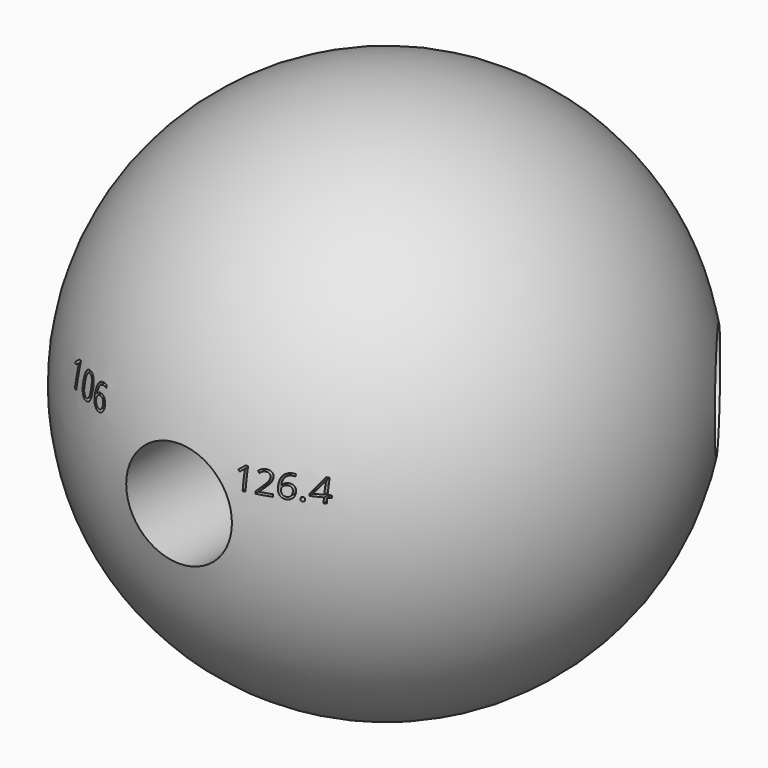
from build123d import *

# Parameters (mm, degrees)
F4_R           = 3.175
F5_DEPTH       = 25.4
F6_ANGLE       = -106
F7_ANGLE       = -127.6
F9_TEXT_SIZE   = 1.9675951787
F9_TEXT_SIZE_2 = 1.7945879437
F10_DEPTH      = 6.35
F12_TEXT_SIZE  = 1.7603325735
F13_DEPTH      = 5.969


# Not quite as in the source:
# - Text() gives the source's letters only with a copy of the font that has no kerning and outlines rounded to 1/6400 em; it was checked with that copy


with BuildPart() as f2:
    # F1 (on Top) → F2 (revolve)
    with BuildSketch(Plane.XY):
        with BuildLine():
            Line((0, -15.875), (0, 15.875))
            ThreePointArc((0, 15.875), (-15.875, 0), (0, -15.875))
        make_face()
    revolve(axis=Axis((0, 0, 0), (0, -1, 0)))

    # F9 (on offset) → F10 (cut)
    with BuildSketch(Plane.XZ.offset(19.05)):
        with Locations((-8.4282197058, 2.6850800496)):
            Text('106', F9_TEXT_SIZE, font='Open Sans', text_align=(TextAlign.LEFT, TextAlign.BOTTOM))
        with Locations((3.1687500887, 1.7594042001)):
            Text('126.4', F9_TEXT_SIZE_2, font='Open Sans', text_align=(TextAlign.LEFT, TextAlign.BOTTOM))
    extrude(amount=-F10_DEPTH, mode=Mode.SUBTRACT)

    # F12 (on offset) → F13 (cut)
    with BuildSketch(Plane(origin=(-18.3120353076, 5.2508916283, 0), x_dir=(-0.2756373558, -0.9612616959, 0), z_dir=(-0.9612616959, 0.2756373558, 0))):
        with Locations((-8.1116128713, 1.9357244018)):
            Text('127.6', F12_TEXT_SIZE, font='Open Sans', text_align=(TextAlign.LEFT, TextAlign.BOTTOM))
    extrude(amount=-F13_DEPTH, mode=Mode.SUBTRACT)


with BuildPart() as f5:
    # F4 (on offset) → F5 (new body)
    with BuildSketch(Plane.XZ.offset(6.35)):
        Circle(F4_R)
    extrude(amount=F5_DEPTH)


with BuildPart() as f6_1:
    # F6: copy of F5
    add(f5.part.rotate(Axis((0, 0, 36.6866141558), (0, 0, 1)), F6_ANGLE))


with BuildPart() as f7_1:
    # F7: copy of F6_1
    add(f6_1.part.rotate(Axis((0, 0, 36.6866141558), (0, 0, 1)), F7_ANGLE))


with BuildPart() as f2_1:
    add(f2.part)

    # F14: cut F5, F7_1, F6_1
    add(f5.part, mode=Mode.SUBTRACT)
    add(f7_1.part, mode=Mode.SUBTRACT)
    add(f6_1.part, mode=Mode.SUBTRACT)


solid = f2_1.part
